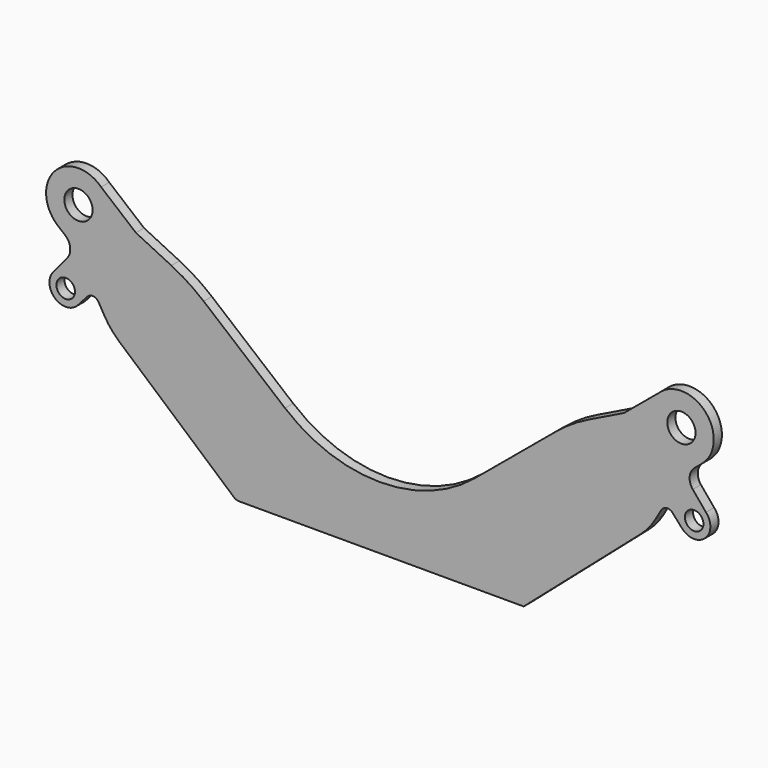
from build123d import *

# Parameters (mm, degrees)
F0_R     = 2
F0_R_2   = 3.05
F1_DEPTH = 2.2
F2_R     = 35
F3_R     = 15
F4_R     = 1.5
F5_R     = 3


with BuildPart() as f1:
    # F0 (on Front) → F1 (new body)
    with BuildSketch(Plane.XZ):
        with BuildLine():
            Line((52.6173001252, 130.7482583531), (41.2109028752, 125.1659909507))
            Line((41.2109028752, 125.1659909507), (20.4584298604, 107.9115033818))
            ThreePointArc((20.4584298604, 107.9115033818), (0, 100.5174507858), (-20.4584298604, 107.9115033818))
            Line((-20.4584298604, 107.9115033818), (-41.2109028752, 125.1659909507))
            Line((-41.2109028752, 125.1659909507), (-52.6173001252, 130.7482583531))
            Line((-52.6173001252, 130.7482583531), (-60.1081627094, 136.9764796956))
            ThreePointArc((-60.1081627094, 136.9764796956), (-70.17561569, 136.6806435954), (-69.4613509604, 126.6342037081))
            Line((-69.4613509604, 126.6342037081), (-65.5419625699, 123.3754577161))
            Line((-65.5419625699, 123.3754577161), (-70.2992250124, 117.6537600959))
            ThreePointArc((-70.2992250124, 117.6537600959), (-70.1188602171, 112.67914718), (-65.1466267703, 112.9162118817))
            Line((-65.1466267703, 112.9162118817), (-61.7026267828, 116.7487230653))
            Line((-61.7026267828, 116.7487230653), (-58.1451833135, 110.6085375713))
            Line((-58.1451833134, 110.6085375713), (-31, 87))
            Line((-31, 87), (31, 87))
            Line((31, 87), (58.1451833134, 110.6085375713))
            Line((58.1451833135, 110.6085375713), (61.7026267828, 116.7487230653))
            Line((61.7026267828, 116.7487230653), (65.1466267703, 112.9162118817))
            ThreePointArc((65.1466267703, 112.9162118817), (70.1188602171, 112.67914718), (70.2992250124, 117.6537600959))
            Line((70.2992250124, 117.6537600959), (65.5419625699, 123.3754577161))
            Line((65.5419625699, 123.3754577161), (69.4613509604, 126.6342037081))
            ThreePointArc((69.4613509604, 126.6342037081), (70.17561569, 136.6806435954), (60.1081627094, 136.9764796956))
            Line((60.1081627094, 136.9764796956), (52.6173001252, 130.7482583531))
        make_face()
        with Locations((-67.7499321664, 115.2556137314)):
            Circle(F0_R, mode=Mode.SUBTRACT)
        with Locations((-65, 132)):
            Circle(F0_R_2, mode=Mode.SUBTRACT)
        with Locations((67.7499321664, 115.2556137314)):
            Circle(F0_R, mode=Mode.SUBTRACT)
        with Locations((65, 132)):
            Circle(F0_R_2, mode=Mode.SUBTRACT)
    extrude(amount=F1_DEPTH)

    # F2
    f2_edges = [f1.edges().sort_by_distance(p)[0] for p in [
        (41.210903, -1.1, 125.165991),
        (-41.210903, -1.1, 125.165991),
    ]]
    fillet(f2_edges, radius=F2_R)

    # F3
    f3_edges = [f1.edges().sort_by_distance(p)[0] for p in [
        (58.145183, -1.1, 110.608538),
        (-58.145183, -1.1, 110.608538),
    ]]
    fillet(f3_edges, radius=F3_R)

    # F4
    f4_edges = [f1.edges().sort_by_distance(p)[0] for p in [
        (-61.702627, -1.1, 116.748723),
        (61.702627, -1.1, 116.748723),
        (-31, -1.1, 87),
    ]]
    fillet(f4_edges, radius=F4_R)

    # F5
    f5_edges = [f1.edges().sort_by_distance(p)[0] for p in [
        (65.541963, -1.1, 123.375458),
        (-65.541963, -1.1, 123.375458),
    ]]
    fillet(f5_edges, radius=F5_R)


solid = f1.part
